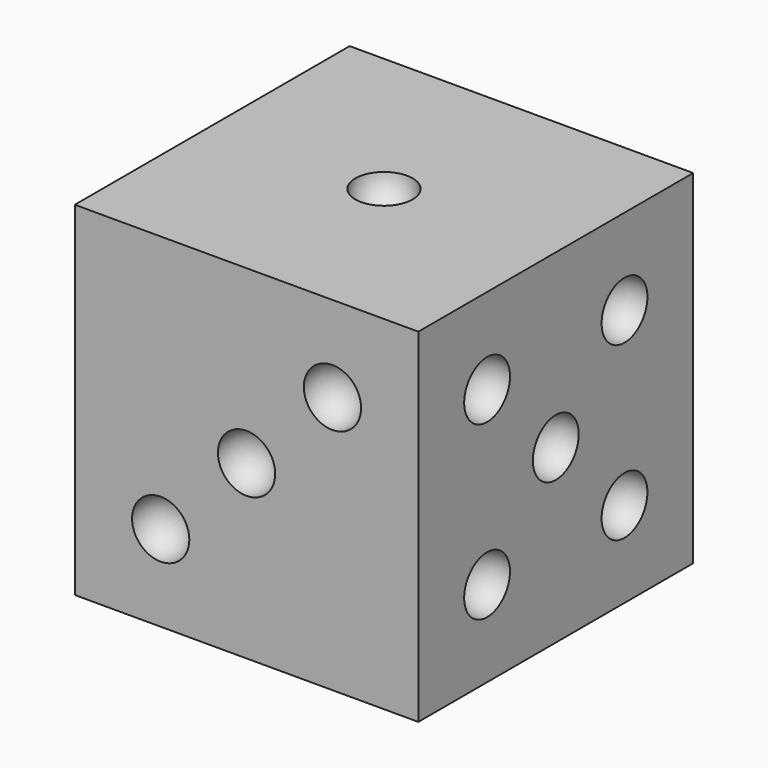
from build123d import *

# Parameters (mm, degrees)
F1_W      = 12
F1_H      = 12
F2_DEPTH  = 12
F3_R      = 1
F4_DEPTH  = 1
F5_R      = 0.99999
F6_R      = 1
F7_DEPTH  = 1
F8_R      = 0.99999
F9_R      = 1
F10_DEPTH = 1
F11_R     = 0.99999
F12_R     = 1
F13_DEPTH = 1
F14_R     = 0.99999


# Not quite as in the source:
# - a fillet or chamfer is up to 0.001 mm smaller than in the source, because OpenCascade refuses the exact size


with BuildPart() as f2:
    # F1 (on offset) → F2 (new body)
    with BuildSketch(Plane.XY.offset(-6)):
        Rectangle(F1_W, F1_H)
    extrude(amount=F2_DEPTH)

    # F3 (on face) → F4 (cut)
    with BuildSketch(Plane.XY.offset(6)):
        Circle(F3_R)
    extrude(amount=-F4_DEPTH, mode=Mode.SUBTRACT)

    # F5 (radius 1 in the source; OpenCascade refuses exactly that, so slightly less here)
    f5_edges = [f2.edges().sort_by_distance(p)[0] for p in [
        (-1, 0, 5),
    ]]
    fillet(f5_edges, radius=F5_R)

    # F6 (on face) → F7 (cut)
    with BuildSketch(Plane.XZ.offset(6)):
        with Locations((3, 3)):
            Circle(F6_R)
        Circle(F6_R)
        with Locations((-3, -3)):
            Circle(F6_R)
    extrude(amount=-F7_DEPTH, mode=Mode.SUBTRACT)

    # F8 (radius 1 in the source; OpenCascade refuses exactly that, so slightly less here)
    f8_edges = [f2.edges().sort_by_distance(p)[0] for p in [
        (2, -5, 3),
        (-1, -5, 0),
        (-4, -5, -3),
    ]]
    fillet(f8_edges, radius=F8_R)

    # F9 (on face) → F10 (cut)
    with BuildSketch(Plane.YZ.offset(6)):
        with Locations((-3, 3)):
            Circle(F9_R)
        Circle(F9_R)
        with Locations((3, 3)):
            Circle(F9_R)
        with Locations((3, -3)):
            Circle(F9_R)
        with Locations((-3, -3)):
            Circle(F9_R)
    extrude(amount=-F10_DEPTH, mode=Mode.SUBTRACT)

    # F11 (radius 1 in the source; OpenCascade refuses exactly that, so slightly less here)
    f11_edges = [f2.edges().sort_by_distance(p)[0] for p in [
        (5, -4, 3),
        (5, -1, 0),
        (5, 2, 3),
        (5, 2, -3),
        (5, -4, -3),
    ]]
    fillet(f11_edges, radius=F11_R)

    # F12 (on face) → F13 (cut)
    with BuildSketch(Plane(origin=(0, 6, 0), x_dir=(-1, 0, 0), z_dir=(0, 1, 0))):
        with Locations((-3, 3)):
            Circle(F12_R)
        with Locations((3, 3)):
            Circle(F12_R)
        with Locations((3, -3)):
            Circle(F12_R)
        with Locations((-3, -3)):
            Circle(F12_R)
    extrude(amount=-F13_DEPTH, mode=Mode.SUBTRACT)

    # F14 (radius 1 in the source; OpenCascade refuses exactly that, so slightly less here)
    f14_edges = [f2.edges().sort_by_distance(p)[0] for p in [
        (4, 5, 3),
        (-2, 5, 3),
        (4, 5, -3),
        (-2, 5, -3),
    ]]
    fillet(f14_edges, radius=F14_R)


solid = f2.part
